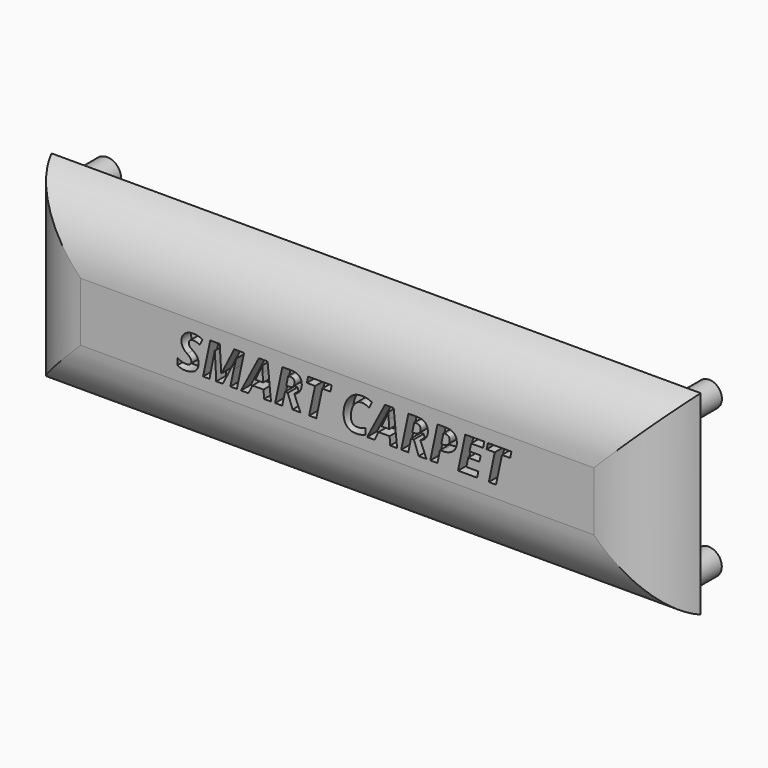
from build123d import *

# Parameters (mm, degrees)
F0_W          = 133.1781893969
F0_H          = 40
F1_DEPTH      = 5
F3_R          = 2.6063085699
F4_DEPTH      = 7.5
F5_R          = 2.8765835579
F6_DEPTH      = 7.5
F7_R          = 2.7014551769
F8_DEPTH      = 7.5
F9_R          = 2.5277062163
F10_DEPTH     = 7.5
F11_T1_DEPTH  = 202.9159221191
F11_T3_DEPTH  = 109.7377327222
F12_TEXT_SIZE = 9.8016708054
F13_DEPTH     = 2.5


# Not quite as in the source:
# - a fillet or chamfer that OpenCascade refuses, or shapes differently, is made with other operations: its cross-section is extruded or revolved along the edge and cut away or added
# - Text() gives the source's letters only with a copy of the font that has no kerning and outlines rounded to 1/6400 em; it was checked with that copy


with BuildPart() as f1:
    # F0 (on Front) → F1 (new body, symmetric)
    with BuildSketch(Plane.XZ):
        Rectangle(F0_W, F0_H)
    extrude(amount=F1_DEPTH, both=True)

    # F3 (on face) → F4 (join, symmetric)
    with BuildSketch(Plane(origin=(0, 5, 0), x_dir=(-1, 0, 0), z_dir=(0, 1, 0))):
        with Locations((-62.3338446021, 15.3954122216)):
            Circle(F3_R)
    extrude(amount=F4_DEPTH, both=True)

    # F5 (on face) → F6 (join, symmetric)
    with BuildSketch(Plane(origin=(0, 5, 0), x_dir=(-1, 0, 0), z_dir=(0, 1, 0))):
        with Locations((61.1956864595, 15.1598416269)):
            Circle(F5_R)
    extrude(amount=F6_DEPTH, both=True)

    # F7 (on face) → F8 (join, symmetric)
    with BuildSketch(Plane(origin=(0, 5, 0), x_dir=(-1, 0, 0), z_dir=(0, 1, 0))):
        with Locations((-62.2093006968, -14.8980282247)):
            Circle(F7_R)
    extrude(amount=F8_DEPTH, both=True)

    # F9 (on face) → F10 (join, symmetric)
    with BuildSketch(Plane(origin=(0, 5, 0), x_dir=(-1, 0, 0), z_dir=(0, 1, 0))):
        with Locations((61.6838186979, -15.0171425194)):
            Circle(F9_R)
    extrude(amount=F10_DEPTH, both=True)

    # F11: fillet of radius 14.7267027305 on 4 edges, made by hand

    # F11_s2 → F11_t1 (cut)
    with BuildSketch(Plane.YZ.offset(-101.4579610595)):
        with BuildLine():
            ThreePointArc((5, 20), (-2.2416831114, 14.6334506967), (-5, 6.0524534556))
            Line((-5, 6.0524534556), (-5, 20))
            Line((-5, 20), (5, 20))
        make_face()
        with BuildLine():
            ThreePointArc((-5, -6.0524534556), (-2.2416831114, -14.6334506967), (5, -20))
            Line((5, -20), (-5, -20))
            Line((-5, -20), (-5, -6.0524534556))
        make_face()
    extrude(amount=F11_T1_DEPTH, mode=Mode.SUBTRACT)

    # F11_s4 → F11_t3 (cut)
    with BuildSketch(Plane.XY.offset(-54.8688663611)):
        with BuildLine():
            ThreePointArc((-66.5890946984, 5), (-61.2225453951, -2.2416831114), (-52.641548154, -5))
            Line((-52.641548154, -5), (-66.5890946984, -5))
            Line((-66.5890946984, -5), (-66.5890946984, 5))
        make_face()
        with BuildLine():
            ThreePointArc((52.641548154, -5), (61.2225453951, -2.2416831114), (66.5890946984, 5))
            Line((66.5890946984, 5), (66.5890946984, -5))
            Line((66.5890946984, -5), (52.641548154, -5))
        make_face()
    extrude(amount=F11_T3_DEPTH, mode=Mode.SUBTRACT)

    # F12 (on face) → F13 (cut, symmetric)
    with BuildSketch(Plane.XZ.offset(5)):
        with Locations((-32.9558667145, -3.5211753566)):
            Text('SMART CARPET', F12_TEXT_SIZE, font='Open Sans', font_style=FontStyle.BOLDITALIC, text_align=(TextAlign.LEFT, TextAlign.BOTTOM))
    extrude(amount=F13_DEPTH, both=True, mode=Mode.SUBTRACT)


solid = f1.part
